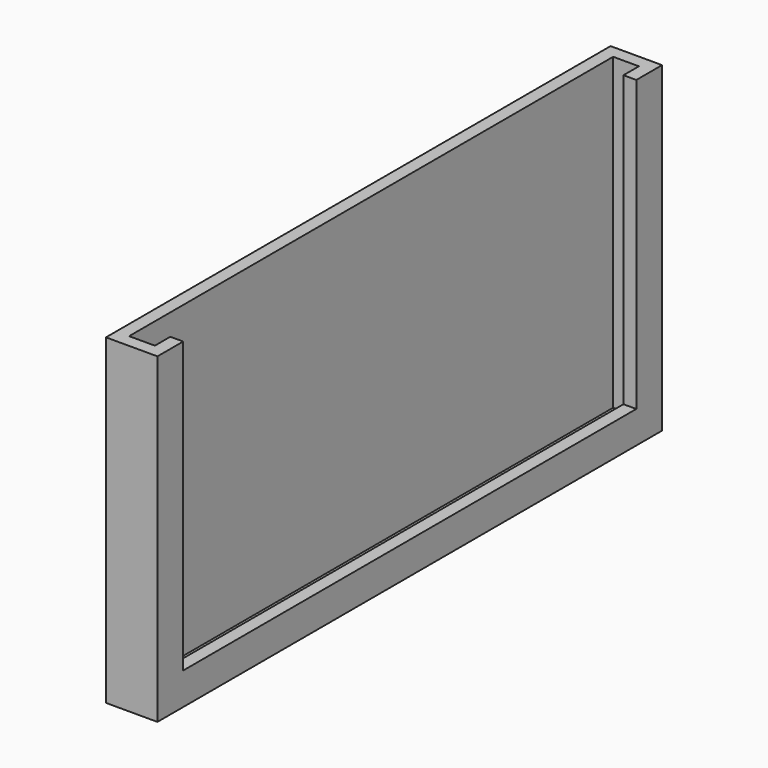
from build123d import *

# Parameters (mm, degrees)
F0_W     = 3.9999993443
F0_H     = 48.9999993443
F0_W_2   = 2
F0_H_2   = 47
F1_DEPTH = 25
F2_W     = 43.9999993443
F2_H     = 22.5
F3_DEPTH = 2
F4_DEPTH = 1


# Not quite as in the source:
# - a feature names something its author has since deleted; it is built from what else it names


with BuildPart() as f1:
    # F0 (on Top) → F1 (new body)
    with BuildSketch(Plane.XY):
        with Locations((1.9999996722, 0)):
            Rectangle(F0_W, F0_H)
        with Locations((1.9999996722, 0)):
            Rectangle(F0_W_2, F0_H_2, mode=Mode.SUBTRACT)
    extrude(amount=F1_DEPTH)

    # F2 (on face) → F3 (cut)
    with BuildSketch(Plane.YZ.offset(3.9999993443)):
        with Locations((0, 13.75)):
            Rectangle(F2_W, F2_H)
    extrude(amount=-F3_DEPTH, mode=Mode.SUBTRACT)

    # F0 (on Top) → F4 (join)
    with BuildSketch(Plane.XY):
        with Locations((1.9999996722, 0)):
            Rectangle(F0_W_2, F0_H_2)
    extrude(amount=F4_DEPTH)


solid = f1.part
